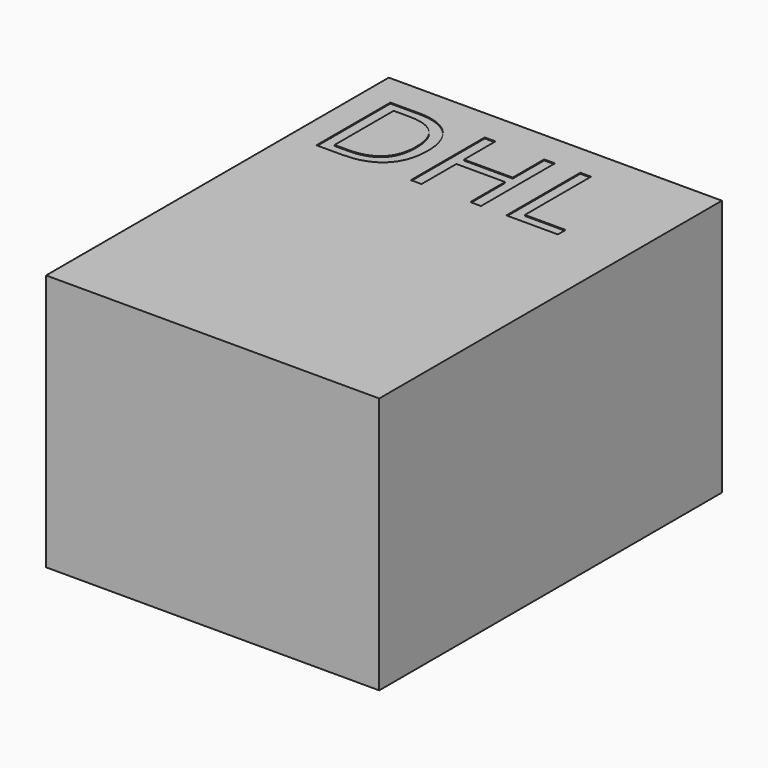
from build123d import *

# Parameters (mm, degrees)
F0_W         = 350
F0_H         = 450
F1_DEPTH     = 270
F3_TEXT_SIZE = 136.028147406
F4_DEPTH     = 1


# Not quite as in the source:
# - Text() gives the source's letters only with a copy of the font that has no kerning and outlines rounded to 1/6400 em; it was checked with that copy


with BuildPart() as f1:
    # F0 (on Top) → F1 (new body)
    with BuildSketch(Plane.XY):
        Rectangle(F0_W, F0_H)
    extrude(amount=F1_DEPTH)

    # F3 (on face) → F4 (cut)
    with BuildSketch(Plane.XY.offset(270)):
        with Locations((-159.6257090569, 94.0982103348)):
            Text('DHL', F3_TEXT_SIZE, font='Open Sans', text_align=(TextAlign.LEFT, TextAlign.BOTTOM))
    extrude(amount=-F4_DEPTH, mode=Mode.SUBTRACT)


solid = f1.part
